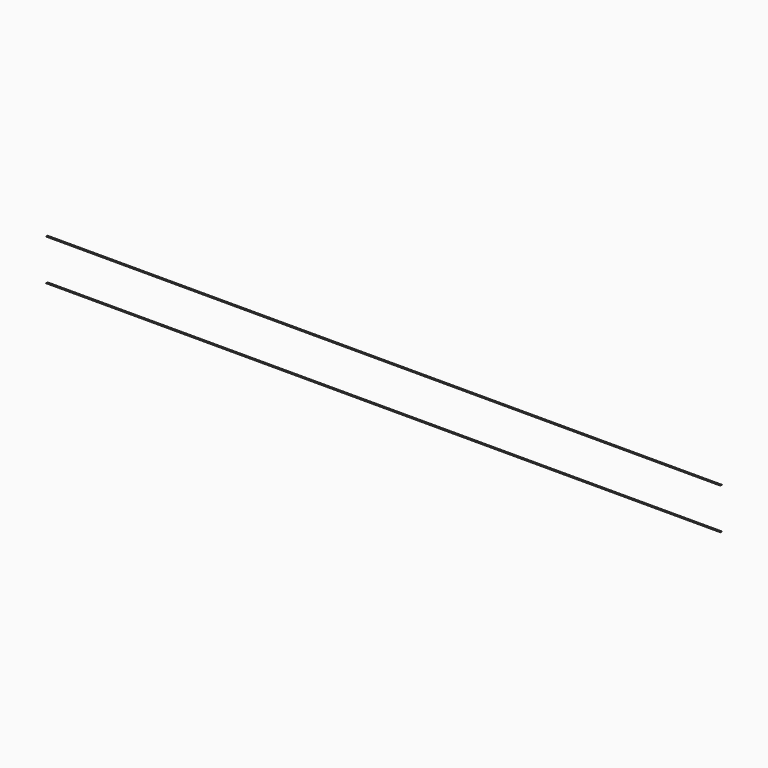
from build123d import *

# Parameters (mm, degrees)
F1_DEPTH = 25.4


with BuildPart() as f1:
    # F0 (on Right) → F1 (new body)
    with BuildSketch(Plane.YZ):
        with BuildLine():
            ThreePointArc((-6.367591743, -4.1314020922), (-6.4033784082, -4.1305748132), (-6.4391650735, -4.1314020922))
            Line((-6.4391650735, -4.1314020922), (-6.367591743, -4.1314020922))
        make_face()
    extrude(amount=F1_DEPTH)


with BuildPart() as f1b:
    # F0 (on Right) → F1, piece 2 (new body)
    with BuildSketch(Plane.YZ):
        with BuildLine():
            ThreePointArc((-6.4391650735, -5.6786441784), (-6.4033784082, -5.6794714575), (-6.367591743, -5.6786441784))
            Line((-6.367591743, -5.6786441784), (-6.4391650735, -5.6786441784))
        make_face()
    extrude(amount=F1_DEPTH)


solid = Compound([f1.part, f1b.part])
